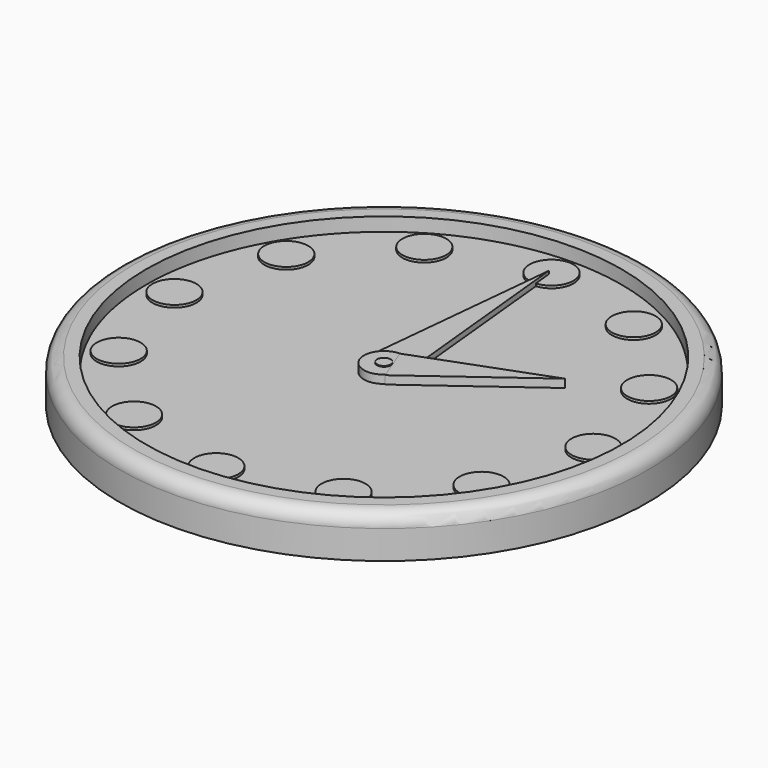
from build123d import *

# Parameters (mm, degrees)
F2_W      = 86.4217877388
F2_H      = 2.7323425747
F4_R      = 5
F5_R      = 2.5029207925
F6_DEPTH  = 3.3
F9_R      = 8.0018065716
F11_DEPTH = 0.9
F12_COUNT = 12
F15_DEPTH = 2
F13_R     = 7.271571706
F16_DEPTH = 3
F18_DEPTH = 3


# Not quite as in the source:
# - the program builds the solid bodies; features that only make, move or delete a surface that nothing else refers to are left out


with BuildPart() as f1:
    # F0 (on Front) → F1 (revolve)
    with BuildSketch(Plane.XZ):
        Polygon((-86.5566954017, 15.4182156548), (-96.1198955774, 15.4182156548), (-96.1198955774, 0), (0, 0), (0, 7.6115243137), (-86.5566954017, 7.6115243137), align=None)
    revolve(axis=Axis((0, 0, 19.0288107842), (0, 0, 1)))

    # F4
    f4_edges = [f1.edges().sort_by_distance(p)[0] for p in [
        (96.119896, 0, 15.418216),
    ]]
    fillet(f4_edges, radius=F4_R)


with BuildPart() as f3:
    # F2 (on Right) → F3 (revolve)
    with BuildSketch(Plane.YZ):
        with Locations((-43.2108938694, 9.1728630941)):
            Rectangle(F2_W, F2_H)
    revolve(axis=Axis((0, 0, 19.0288107842), (0, 0, 1)))

    # F5 (on face) → F6 (join)
    with BuildSketch(Plane.XY.offset(10.5390343815)):
        Circle(F5_R)
    extrude(amount=F6_DEPTH)

    # F9 (on face) → F11 (join)
    with BuildSketch(Plane.XY.offset(10.5390343815)):
        with Locations((0, 76.2884691358)):
            Circle(F9_R)
    extrude(amount=F11_DEPTH)


with BuildPart() as f12_1:
    # F12: instance of F3
    add(f3.part.rotate(Axis((0, 0, 36.9842015207), (0, 0, 1)), 1 * 360 / F12_COUNT))


with BuildPart() as f12_2:
    # F12: instance of F3
    add(f3.part.rotate(Axis((0, 0, 36.9842015207), (0, 0, 1)), 2 * 360 / F12_COUNT))


with BuildPart() as f12_3:
    # F12: instance of F3
    add(f3.part.rotate(Axis((0, 0, 36.9842015207), (0, 0, 1)), 3 * 360 / F12_COUNT))


with BuildPart() as f12_4:
    # F12: instance of F3
    add(f3.part.rotate(Axis((0, 0, 36.9842015207), (0, 0, 1)), 4 * 360 / F12_COUNT))


with BuildPart() as f12_5:
    # F12: instance of F3
    add(f3.part.rotate(Axis((0, 0, 36.9842015207), (0, 0, 1)), 5 * 360 / F12_COUNT))


with BuildPart() as f12_6:
    # F12: instance of F3
    add(f3.part.rotate(Axis((0, 0, 36.9842015207), (0, 0, 1)), 6 * 360 / F12_COUNT))


with BuildPart() as f12_7:
    # F12: instance of F3
    add(f3.part.rotate(Axis((0, 0, 36.9842015207), (0, 0, 1)), 7 * 360 / F12_COUNT))


with BuildPart() as f12_8:
    # F12: instance of F3
    add(f3.part.rotate(Axis((0, 0, 36.9842015207), (0, 0, 1)), 8 * 360 / F12_COUNT))


with BuildPart() as f12_9:
    # F12: instance of F3
    add(f3.part.rotate(Axis((0, 0, 36.9842015207), (0, 0, 1)), 9 * 360 / F12_COUNT))


with BuildPart() as f12_10:
    # F12: instance of F3
    add(f3.part.rotate(Axis((0, 0, 36.9842015207), (0, 0, 1)), 10 * 360 / F12_COUNT))


with BuildPart() as f12_11:
    # F12: instance of F3
    add(f3.part.rotate(Axis((0, 0, 36.9842015207), (0, 0, 1)), 11 * 360 / F12_COUNT))


with BuildPart() as f15:
    # F14 (on face) → F15 (new body)
    with BuildSketch(Plane.XY.offset(10.5390343815)):
        Polygon((7.5312675908, 0), (0, 75.0378370285), (-7.4763009325, 0), align=None)
    extrude(amount=F15_DEPTH)


with BuildPart() as f16:
    # F13 (on face) → F16 (new body)
    with BuildSketch(Plane.XY.offset(10.5390343815)):
        Circle(F13_R)
    extrude(amount=F16_DEPTH)


with BuildPart() as f18:
    # F17 (on face) → F18 (new body)
    with BuildSketch(Plane.XY.offset(10.5390343815)):
        Polygon((46.300817281, 24.5123598725), (0, 7.2536570951), (5.0300061703, -5.752901081), align=None)
    extrude(amount=F18_DEPTH)


solid = Compound([f1.part, f3.part, f12_1.part, f12_2.part, f12_3.part, f12_4.part, f12_5.part, f12_6.part, f12_7.part, f12_8.part, f12_9.part, f12_10.part, f12_11.part, f15.part, f16.part, f18.part])
